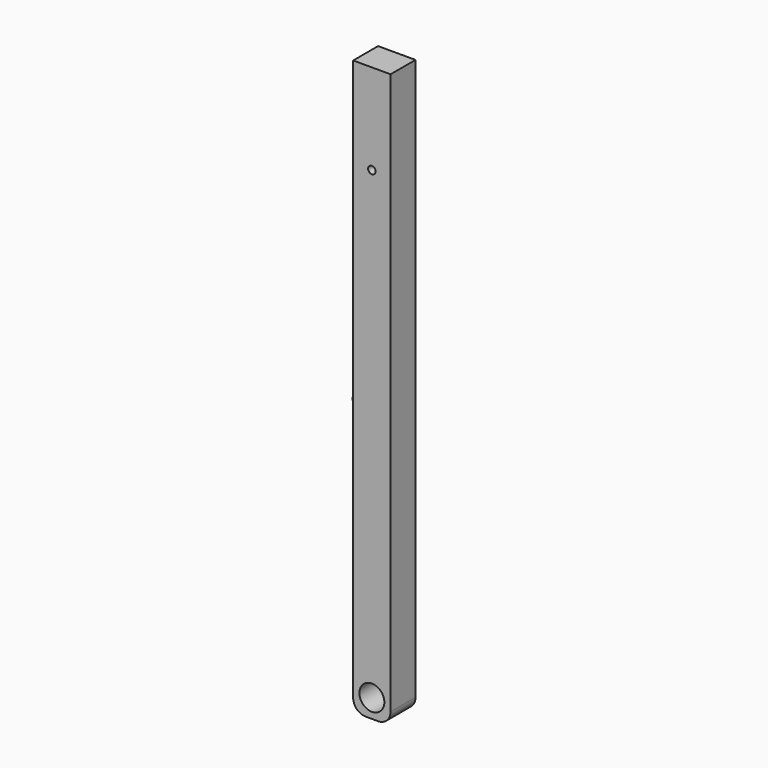
from build123d import *

# Parameters (mm, degrees)
F0_R      = 10
F1_DEPTH  = 25
F2_W      = 20
F2_H      = 24
F3_DEPTH  = 12.5
F4_SIZE   = 12.49999
F5_R      = 2
F9_R      = 3
F10_DEPTH = 25


# Not quite as in the source:
# - a fillet or chamfer is up to 0.001 mm smaller than in the source, because OpenCascade refuses the exact size


with BuildPart() as f1:
    # F0 (on Front) → F1 (new body)
    with BuildSketch(Plane.XZ):
        with BuildLine():
            ThreePointArc((-15, -5), (-12.0710678119, -12.0710678119), (-5, -15))
            Line((-5, -15), (5, -15))
            ThreePointArc((5, -15), (12.0710678119, -12.0710678119), (15, -5))
            Line((15, -5), (15, 15))
            Line((15, 15), (15, 445))
            Line((15, 445), (-15, 445))
            Line((-15, 445), (-15, 15))
            Line((-15, 15), (-15, -5))
        make_face()
        Circle(F0_R, mode=Mode.SUBTRACT)
    extrude(amount=F1_DEPTH)

    # F2 (on face) → F3 (cut)
    with BuildSketch(Plane(origin=(-15, 0, 0), x_dir=(0, -1, 0), z_dir=(-1, 0, 0))):
        with Locations((12.5, 410)):
            Rectangle(F2_W, F2_H)
    extrude(amount=-F3_DEPTH, mode=Mode.SUBTRACT)

    # F4 (size 12.5 in the source; OpenCascade refuses exactly that, so slightly less here)
    f4_edges = [f1.edges().sort_by_distance(p)[0] for p in [
        (-2.5, -12.5, 422),
    ]]
    chamfer(f4_edges, length=F4_SIZE)

    # F8: sweep along a path in F7
    with BuildLine(Plane.XY.offset(201)) as f8_path:
        ThreePointArc((-15, -18.75), (-21.25, -12.5), (-15, -6.25))
    # F5 (on face) → F8 (sweep)
    with BuildSketch(Plane(origin=(-15, 0, 0), x_dir=(0, -1, 0), z_dir=(-1, 0, 0))):
        with Locations((6.25, 201)):
            Circle(F5_R)
    sweep(path=f8_path.line)

    # F9 (on face) → F10 (cut, through all)
    with BuildSketch(Plane(origin=(0, 0, 0), x_dir=(-1, 0, 0), z_dir=(0, 1, 0))):
        with Locations((0, 372.5)):
            Circle(F9_R)
    extrude(amount=-F10_DEPTH, mode=Mode.SUBTRACT)


solid = f1.part
